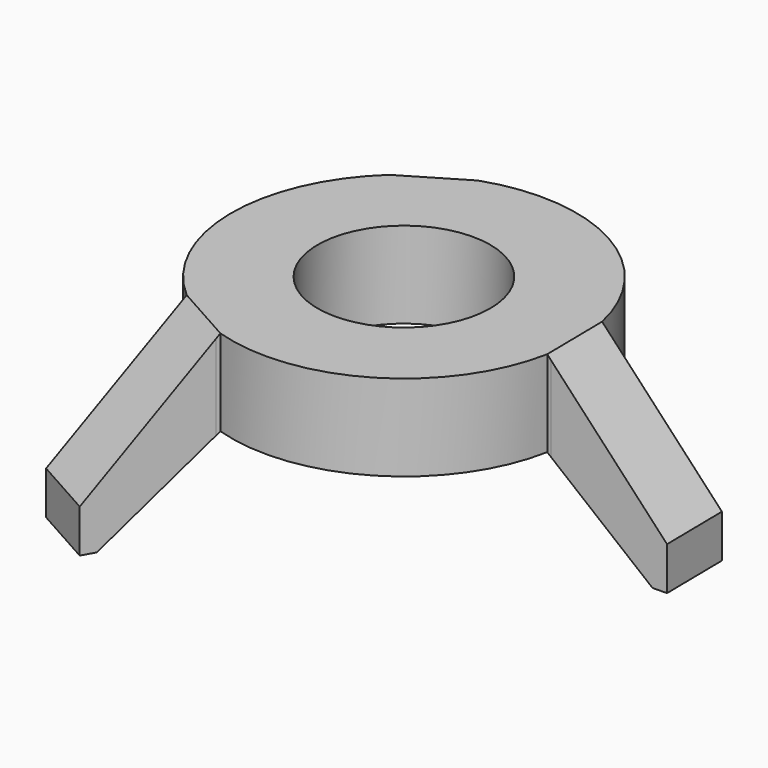
from build123d import *

# Parameters (mm, degrees)
F0_R     = 76.2
F1_DEPTH = 152.4
F2_R     = 76.2
F3_DEPTH = 76.2
F5_DEPTH = 76.2
F7_DEPTH = 76.2
F9_DEPTH = 76.2


with BuildPart() as f1:
    # F0 (on Top) → F1 (new body)
    with BuildSketch(Plane.XY):
        with BuildLine():
            ThreePointArc((-102.8660584411, 112.447027621), (-77.9844038606, 130.9358344935), (-49.8762557284, 144.0073578485))
            Line((-49.8762557284, 144.0073578485), (-51.4895025042, 146.7159996073))
            Line((-51.4895025042, 146.7159996073), (-103.4791050779, 234.0065559363))
            Line((-103.4791050779, 234.0065559363), (-156.4689077906, 202.4462257088))
            Line((-156.4689077906, 202.4462257088), (-104.4793052169, 115.1556693797))
            Line((-104.4793052169, 115.1556693797), (-102.8660584411, 112.447027621))
        make_face()
        with BuildLine():
            ThreePointArc((149.6603896108, -28.7667826068), (151.7135514328, -14.4484709107), (152.4, 0))
            ThreePointArc((152.4, 0), (151.5011019534, 16.5280400202), (148.8150117204, 32.8611059867))
            ThreePointArc((148.8150117204, 32.8611059867), (74.4015570068, 133.004392089), (-49.8762557284, 144.0073578485))
            ThreePointArc((-49.8762557284, 144.0073578485), (-77.9844038606, 130.9358344935), (-102.8660584411, 112.447027621))
            ThreePointArc((-102.8660584411, 112.447027621), (-152.3859608674, -2.0685575955), (-99.7759023645, -115.1977834307))
            ThreePointArc((-99.7759023645, -115.1977834307), (-74.4015570068, -133.004392089), (-45.9489532793, -145.3081336077))
            ThreePointArc((-45.9489532793, -145.3081336077), (78.0031225642, -130.9246839608), (149.6603896108, -28.7667826068))
        make_face()
        Circle(F0_R, mode=Mode.SUBTRACT)
        with BuildLine():
            Line((-47.4880824642, -148.0595671774), (-45.9489532793, -145.3081336077))
            ThreePointArc((-45.9489532793, -145.3081336077), (-74.4015570068, -133.004392089), (-99.7759023645, -115.1977834307))
            Line((-99.7759023645, -115.1977834307), (-101.3150315494, -117.9492170005))
            Line((-101.3150315494, -117.9492170005), (-150.916069554, -206.6188117265))
            Line((-150.916069554, -206.6188117265), (-97.0891204688, -236.7291619034))
            Line((-97.0891204688, -236.7291619034), (-47.4880824642, -148.0595671774))
        make_face()
        with BuildLine():
            ThreePointArc((148.8150117204, 32.8611059867), (151.5011019534, 16.5280400202), (152.4, 0))
            ThreePointArc((152.4, 0), (151.7135514328, -14.4484709107), (149.6603896108, -28.7667826068))
            Line((149.6603896108, -28.7667826068), (152.8045340537, -28.7667826068))
            Line((152.8045340537, -28.7667826068), (254.3951746319, -27.3877442098))
            Line((254.3951746319, -27.3877442098), (253.5580282594, 34.2829361947))
            Line((253.5580282594, 34.2829361947), (151.9673876811, 32.9038977977))
            Line((151.9673876811, 32.9038977977), (148.8150117204, 32.8611059867))
        make_face()
    extrude(amount=F1_DEPTH)

    # F2 (on face) → F3 (cut)
    with BuildSketch(Plane(origin=(0, 0, 0), x_dir=(1, 0, 0), z_dir=(0, 0, -1))):
        with BuildLine():
            ThreePointArc((148.8150117204, -32.8611059867), (151.5011019534, -16.5280400202), (152.4, 0))
            ThreePointArc((152.4, 0), (151.7135514328, 14.4484709107), (149.6603896108, 28.7667826068))
            ThreePointArc((149.6603896108, 28.7667826068), (78.0031225642, 130.9246839608), (-45.9489532793, 145.3081336077))
            ThreePointArc((-45.9489532793, 145.3081336077), (-74.4015570068, 133.004392089), (-99.7759023645, 115.1977834307))
            ThreePointArc((-99.7759023645, 115.1977834307), (-152.3859608674, 2.0685575955), (-102.8660584411, -112.447027621))
            ThreePointArc((-102.8660584411, -112.447027621), (-77.9844038606, -130.9358344935), (-49.8762557284, -144.0073578485))
            ThreePointArc((-49.8762557284, -144.0073578485), (74.4015570068, -133.004392089), (148.8150117204, -32.8611059867))
        make_face()
        Circle(F2_R, mode=Mode.SUBTRACT)
        Circle(F2_R)
    extrude(amount=-F3_DEPTH, mode=Mode.SUBTRACT)

    # F4 (on face) → F5 (cut)
    with BuildSketch(Plane(origin=(-0.4185731863, 30.8353402022, 0), x_dir=(-0.9999078797, -0.0135732126, 0), z_dir=(-0.0135732126, 0.9999078797, 0))):
        Polygon((-254, 38.1), (-149.2473336147, 152.4), (-254, 152.4), align=None)
        Polygon((-149.2473336147, 0), (-149.2473336147, 76.2), (-241.3, 0), align=None)
    extrude(amount=-F5_DEPTH, mode=Mode.SUBTRACT)

    # F6 (on face) → F7 (cut)
    with BuildSketch(Plane(origin=(-26.4949013563, -15.7801651138, 0), x_dir=(0.5117086867, -0.859159019, 0), z_dir=(-0.859159019, -0.5117086867, 0))):
        Polygon((-254, 38.1), (-149.2473336147, 152.4), (-254, 152.4), align=None)
        Polygon((-149.2473336147, 0), (-149.2473336147, 76.2), (-241.3, 0), align=None)
    extrude(amount=-F7_DEPTH, mode=Mode.SUBTRACT)

    # F8 (on face) → F9 (cut)
    with BuildSketch(Plane(origin=(26.9134745426, -15.0551750885, 0), x_dir=(0.488199193, 0.8727322316, 0), z_dir=(0.8727322316, -0.488199193, 0))):
        Polygon((-254, 38.1), (-149.2473336147, 152.4), (-254, 152.4), align=None)
        Polygon((-149.2473336147, 0), (-149.2473336147, 76.2), (-241.3, 0), align=None)
    extrude(amount=-F9_DEPTH, mode=Mode.SUBTRACT)


solid = f1.part
